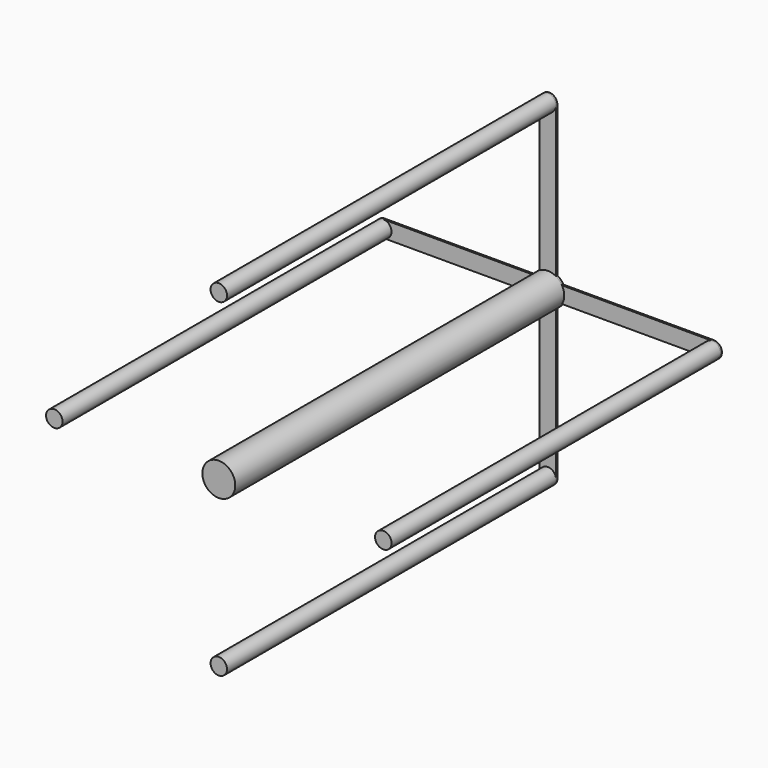
from build123d import *

# Parameters (mm, degrees)
F0_R     = 10
F1_DEPTH = 250
F0_R_2   = 5
F3_DEPTH = 1.06
F4_R     = 6.35
F5_DEPTH = 50


with BuildPart() as f1:
    # F0 (on Front) → F1 (new body)
    with BuildSketch(Plane.XZ):
        Circle(F0_R)
    extrude(amount=F1_DEPTH)


with BuildPart() as f1b:
    # F0 (on Front) → F1, piece 2 (new body)
    with BuildSketch(Plane.XZ):
        with Locations((-100, 0)):
            Circle(F0_R_2)
    extrude(amount=F1_DEPTH)


with BuildPart() as f1c:
    # F0 (on Front) → F1, piece 3 (new body)
    with BuildSketch(Plane.XZ):
        with Locations((0, -100)):
            Circle(F0_R_2)
    extrude(amount=F1_DEPTH)


with BuildPart() as f1d:
    # F0 (on Front) → F1, piece 4 (new body)
    with BuildSketch(Plane.XZ):
        with Locations((100, 0)):
            Circle(F0_R_2)
    extrude(amount=F1_DEPTH)


with BuildPart() as f1e:
    # F0 (on Front) → F1, piece 5 (new body)
    with BuildSketch(Plane.XZ):
        with Locations((0, 100)):
            Circle(F0_R_2)
    extrude(amount=F1_DEPTH)


with BuildPart() as f3:
    # F2 (on face) → F3 (new body)
    with BuildSketch(Plane(origin=(0, 0, 0), x_dir=(-1, 0, 0), z_dir=(0, 1, 0))):
        with BuildLine():
            ThreePointArc((8.6602540378, -5), (9.6592582629, -2.588190451), (10, 0))
            ThreePointArc((10, 0), (9.6592582629, 2.588190451), (8.6602540378, 5))
            ThreePointArc((8.6602540378, 5), (7.0710678119, 7.0710678119), (5, 8.6602540378))
            ThreePointArc((5, 8.6602540378), (0, 10), (-5, 8.6602540378))
            ThreePointArc((-5, 8.6602540378), (-7.0710678119, 7.0710678119), (-8.6602540378, 5))
            ThreePointArc((-8.6602540378, 5), (-10, 0), (-8.6602540378, -5))
            ThreePointArc((-8.6602540378, -5), (-7.0710678119, -7.0710678119), (-5, -8.6602540378))
            ThreePointArc((-5, -8.6602540378), (0, -10), (5, -8.6602540378))
            ThreePointArc((5, -8.6602540378), (7.0710678119, -7.0710678119), (8.6602540378, -5))
        make_face()
        with BuildLine():
            ThreePointArc((8.6602540378, 5), (9.6592582629, 2.588190451), (10, 0))
            ThreePointArc((10, 0), (9.6592582629, -2.588190451), (8.6602540378, -5))
            Line((8.6602540378, -5), (100, -5))
            ThreePointArc((100, -5), (95, 0), (100, 5))
            Line((100, 5), (8.6602540378, 5))
        make_face()
        with BuildLine():
            ThreePointArc((-5, 8.6602540378), (0, 10), (5, 8.6602540378))
            Line((5, 8.6602540378), (5, 100))
            ThreePointArc((5, 100), (0, 95), (-5, 100))
            Line((-5, 100), (-5, 8.6602540378))
        make_face()
        with BuildLine():
            ThreePointArc((105, 0), (103.5355339059, 3.5355339059), (100, 5))
            ThreePointArc((100, 5), (95, 0), (100, -5))
            ThreePointArc((100, -5), (103.5355339059, -3.5355339059), (105, 0))
        make_face()
        with BuildLine():
            Line((5, -100), (5, -8.6602540378))
            ThreePointArc((5, -8.6602540378), (0, -10), (-5, -8.6602540378))
            Line((-5, -8.6602540378), (-5, -100))
            ThreePointArc((-5, -100), (0, -95), (5, -100))
        make_face()
        with BuildLine():
            ThreePointArc((-5, 100), (0, 95), (5, 100))
            ThreePointArc((5, 100), (0, 105), (-5, 100))
        make_face()
        with BuildLine():
            ThreePointArc((-5, -100), (0, -105), (5, -100))
            ThreePointArc((5, -100), (0, -95), (-5, -100))
        make_face()
        with BuildLine():
            ThreePointArc((-8.6602540378, -5), (-10, 0), (-8.6602540378, 5))
            Line((-8.6602540378, 5), (-100, 5))
            ThreePointArc((-100, 5), (-96.4644660941, 3.5355339059), (-95, 0))
            ThreePointArc((-95, 0), (-96.4644660941, -3.5355339059), (-100, -5))
            Line((-100, -5), (-8.6602540378, -5))
        make_face()
        with BuildLine():
            ThreePointArc((-95, 0), (-96.4644660941, 3.5355339059), (-100, 5))
            ThreePointArc((-100, 5), (-105, 0), (-100, -5))
            ThreePointArc((-100, -5), (-96.4644660941, -3.5355339059), (-95, 0))
        make_face()
    extrude(amount=F3_DEPTH)

    # F4 (on face) → F5 (cut)
    with BuildSketch(Plane(origin=(0, 1.06, 0), x_dir=(-1, 0, 0), z_dir=(0, 1, 0))):
        Circle(F4_R)
    extrude(amount=-F5_DEPTH, mode=Mode.SUBTRACT)


solid = Compound([f1.part, f1b.part, f1c.part, f1d.part, f1e.part, f3.part])
